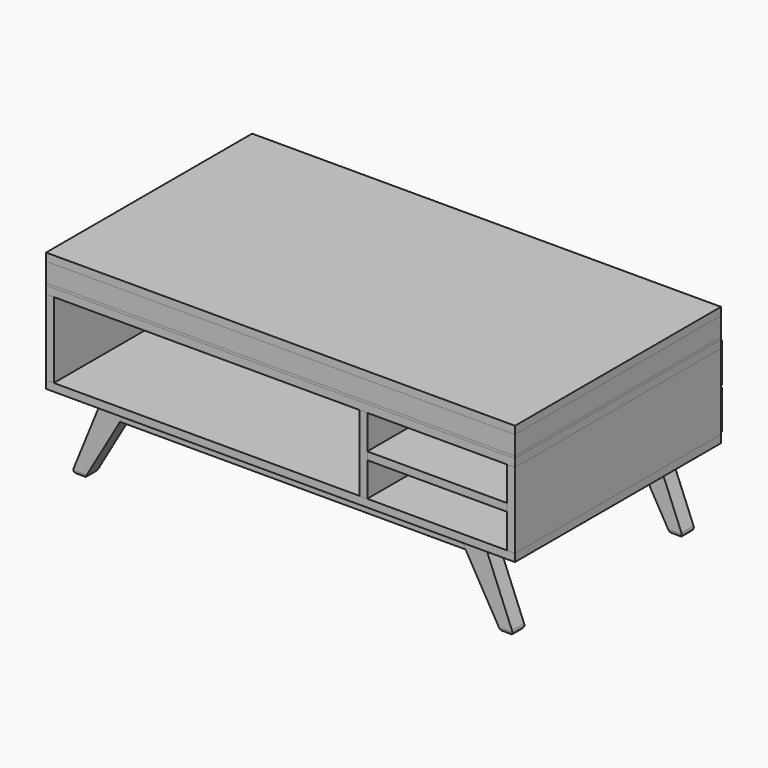
from build123d import *

# Parameters (mm, degrees)
F1_DEPTH       = 340.5
F1_DEPTH_BACK  = 340.5
F2_DEPTH       = 340.5
F2_DEPTH_BACK  = 340.5
F0_W           = 20.5
F0_H           = 200
F3_DEPTH       = 340.5
F3_DEPTH_BACK  = 340.5
F6_DEPTH       = 40
F7_R           = 10
F7_2_R         = 10
F8_DEPTH       = 40
F10_W          = 46.1880215352
F10_H          = 40
F11_DEPTH      = 520
F12_W          = 7
F12_H          = 96.75
F13_DEPTH      = 20
F14_W          = 1240
F14_H          = 681
F14_W_2        = 1230
F14_H_2        = 671
F14_W_3        = 1199
F14_H_3        = 640
F15_DEPTH      = 6
F16_W          = 898.5
F16_H          = 637
F17_DEPTH      = 3
F16_W_2        = 297.5
F18_DEPTH      = 3
F19_DEPTH      = 50
F20_W          = 1240
F20_H          = 681
F21_DEPTH      = 20.5
F23_DEPTH      = 370
F0_W_2         = 370
F0_H_2         = 20.5
F24_DEPTH      = 19.5
F24_DEPTH_BACK = 340.5


# Not quite as in the source:
# - a feature names something its author has since deleted; it is built from what else it names


with BuildPart() as f1:
    # F0 (on Front) → F1 (new body, two sides)
    with BuildSketch(Plane.XZ) as f1_sk:
        Polygon((-599.5, -220.5), (-620, -220.5), (-620, -241), (620, -241), (620, -220.5), (599.5, -220.5), (229.5, -220.5), (209, -220.5), align=None)
    extrude(amount=F1_DEPTH)
    extrude(f1_sk.sketch, amount=-F1_DEPTH_BACK)


with BuildPart() as f2:
    # F0 (on Front) → F2 (new body, two sides)
    with BuildSketch(Plane.XZ) as f2_sk:
        Polygon((229.5, -20.5), (209, -20.5), (209, -220.5), (229.5, -220.5), (229.5, -130.75), (229.5, -110.25), align=None)
    extrude(amount=F2_DEPTH)
    extrude(f2_sk.sketch, amount=-F2_DEPTH_BACK)


with BuildPart() as f2b:
    # F0 (on Front) → F2, piece 2 (new body, two sides)
    with BuildSketch(Plane.XZ) as f2_2_sk:
        with Locations((-609.75, -120.5)):
            Rectangle(F0_W, F0_H)
    extrude(amount=F2_DEPTH)
    extrude(f2_2_sk.sketch, amount=-F2_DEPTH_BACK)


with BuildPart() as f2c:
    # F0 (on Front) → F2, piece 3 (new body, two sides)
    with BuildSketch(Plane.XZ) as f2_3_sk:
        Polygon((620, -220.5), (620, -20.5), (599.5, -20.5), (599.5, -110.25), (599.5, -130.75), (599.5, -220.5), align=None)
    extrude(amount=F2_DEPTH)
    extrude(f2_3_sk.sketch, amount=-F2_DEPTH_BACK)


with BuildPart() as f3:
    # F0 (on Front) → F3 (new body, two sides)
    with BuildSketch(Plane.XZ) as f3_sk:
        Polygon((620, 0), (-620, 0), (-620, -20.5), (-599.5, -20.5), (209, -20.5), (229.5, -20.5), (599.5, -20.5), (620, -20.5), align=None)
    extrude(amount=F3_DEPTH)
    extrude(f3_sk.sketch, amount=-F3_DEPTH_BACK)


with BuildPart() as f6:
    # F5 (on offset) → F6 (new body)
    with BuildSketch(Plane.XZ.offset(260)):
        Polygon((-433.8045381863, -241), (-503.0865704891, -241), (-585.3589838486, -443.5), (-550.7179676972, -443.5), (-456.8985489539, -281), align=None)
    extrude(amount=F6_DEPTH)

    # F7
    f7_edges = [f6.edges().sort_by_distance(p)[0] for p in [
        (-568.038476, -300, -443.5),
        (-550.717968, -280, -443.5),
        (-568.038476, -260, -443.5),
        (-585.358984, -280, -443.5),
    ]]
    fillet(f7_edges, radius=F7_R)


with BuildPart() as f6b:
    # F5 (on offset) → F6, piece 2 (new body)
    with BuildSketch(Plane.XZ.offset(260)):
        Polygon((503.0865704891, -241), (433.8045381863, -241), (456.8985489539, -281), (550.7179676972, -443.5), (585.3589838486, -443.5), align=None)
    extrude(amount=F6_DEPTH)

    # F7#2
    f7_2_edges = [f6b.edges().sort_by_distance(p)[0] for p in [
        (568.038476, -300, -443.5),
        (550.717968, -280, -443.5),
        (568.038476, -260, -443.5),
        (585.358984, -280, -443.5),
    ]]
    fillet(f7_2_edges, radius=F7_2_R)


with BuildPart() as f8:
    # F5 (on offset) → F8 (new body)
    with BuildSketch(Plane.XZ.offset(260)):
        Polygon((433.8045381863, -241), (-433.8045381863, -241), (-456.8985489539, -281), (456.8985489539, -281), align=None)
    extrude(amount=F8_DEPTH)


with BuildPart() as f9_1:
    # F9: instance of F6
    add(f6.part.mirror(Plane.XZ))


with BuildPart() as f9_2:
    # F9: instance of F6b
    add(f6b.part.mirror(Plane.XZ))


with BuildPart() as f9_3:
    # F9: instance of F8
    add(f8.part.mirror(Plane.XZ))


with BuildPart() as f11:
    # F10 (on face) → F11 (new body, through all)
    with BuildSketch(Plane.XZ.offset(260)):
        with Locations((479.9925597215, -261)):
            Rectangle(F10_W, F10_H)
    extrude(amount=-F11_DEPTH)


with BuildPart() as f11b:
    # F10 (on face) → F11, piece 2 (new body, through all)
    with BuildSketch(Plane.XZ.offset(260)):
        with Locations((-479.9925597215, -261)):
            Rectangle(F10_W, F10_H)
    extrude(amount=-F11_DEPTH)


with BuildPart() as f13:
    # F12 (on face) → F13 (new body)
    with BuildSketch(Plane(origin=(0, 340.5, 0), x_dir=(-1, 0, 0), z_dir=(0, 1, 0))):
        with Locations((-603, -68.875)):
            Rectangle(F12_W, F12_H)
        Polygon((-222.5, -117.25), (-222.5, -13.5), (-606.5, -13.5), (-606.5, -20.5), (-599.5, -20.5), (-599.5, -117.25), align=None)
    extrude(amount=F13_DEPTH)


with BuildPart() as f13b:
    # F12 (on face) → F13, piece 2 (new body)
    with BuildSketch(Plane(origin=(0, 340.5, 0), x_dir=(-1, 0, 0), z_dir=(0, 1, 0))):
        with Locations((-603, -172.125)):
            Rectangle(F12_W, F12_H)
        Polygon((-222.5, -123.75), (-599.5, -123.75), (-599.5, -220.5), (-606.5, -220.5), (-606.5, -227.5), (-222.5, -227.5), align=None)
    extrude(amount=F13_DEPTH)


with BuildPart() as f15:
    # F14 (on face) → F15 (new body)
    with BuildSketch(Plane.XY):
        Rectangle(F14_W, F14_H)
        Rectangle(F14_W_2, F14_H_2, mode=Mode.SUBTRACT)
        Rectangle(F14_W_2, F14_H_2)
        Rectangle(F14_W_3, F14_H_3, mode=Mode.SUBTRACT)
    extrude(amount=F15_DEPTH)


with BuildPart() as f17:
    # F16 (on face) → F17 (new body)
    with BuildSketch(Plane.XY):
        with Locations((-148.75, 0)):
            Rectangle(F16_W, F16_H)
    extrude(amount=F17_DEPTH)


with BuildPart() as f18:
    # F16 (on face) → F18 (new body, through all)
    with BuildSketch(Plane.XY):
        with Locations((449.25, 0)):
            Rectangle(F16_W_2, F16_H)
    extrude(amount=F18_DEPTH)


with BuildPart() as f19:
    # F19 (new): a face of the model
    f19_faces = [f15.part.faces().sort_by_distance(p)[0] for p in [
        (-613.646946667, 0, 6),
    ]]
    extrude(f19_faces, amount=F19_DEPTH)


with BuildPart() as f21:
    # F20 (on face) → F21 (new body)
    with BuildSketch(Plane.XY.offset(56)):
        Rectangle(F20_W, F20_H)
    extrude(amount=F21_DEPTH)


with BuildPart() as f23:
    # F22 (on face) → F23 (new body, through all)
    with BuildSketch(Plane.YZ.offset(229.5)):
        Polygon((40, -20.5), (19.5, -20.5), (19.5, -130.75), (19.5, -220.5), (40, -220.5), (40, -130.75), align=None)
    extrude(amount=F23_DEPTH)


with BuildPart() as f24:
    # F0 (on Front) → F24 (new body, two sides)
    with BuildSketch(Plane.XZ) as f24_sk:
        with Locations((414.5, -120.5)):
            Rectangle(F0_W_2, F0_H_2)
    extrude(amount=-F24_DEPTH)
    extrude(f24_sk.sketch, amount=F24_DEPTH_BACK)


solid = Compound([f1.part, f2.part, f2b.part, f2c.part, f3.part, f6.part, f6b.part, f8.part, f9_1.part, f9_2.part, f9_3.part, f11.part, f11b.part, f13.part, f13b.part, f15.part, f17.part, f18.part, f19.part, f21.part, f23.part, f24.part])
